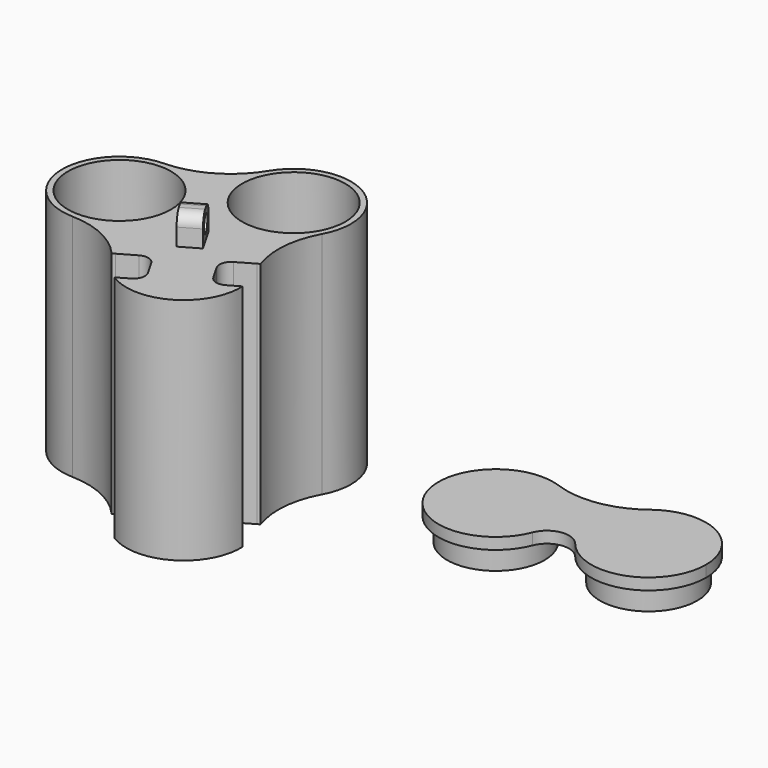
from build123d import *

# Parameters (mm, degrees)
F0_R     = 11.43
F1_DEPTH = 50.8
F2_R     = 11.43
F3_DEPTH = 48.26
F5_DEPTH = 6.35
F6_R     = 11.303
F7_DEPTH = 2.54
F8_R     = 10.795
F8_R_2   = 10.16
F9_DEPTH = 5.08
F10_R    = 2.54
F12_D    = 3.81


# Not quite as in the source:
# - a feature names something its author has since deleted; it is built from what else it names


with BuildPart() as f1:
    # F0 (on Top) → F1 (new body)
    with BuildSketch(Plane.XY):
        with BuildLine():
            ThreePointArc((-26.6880410914, -27.9366493299), (-17.5198893886, -24.3227590811), (-13.696455988, -15.239997089))
            ThreePointArc((-13.696455988, -15.239997089), (-17.5198098165, -6.1573128632), (-26.687818625, -2.5433397409))
            ThreePointArc((-26.687818625, -2.5433397409), (-39.0964559875, -15.2398858265), (-26.6880410914, -27.9366493299))
        make_face()
        with Locations((-26.396455988, -15.239997089)):
            Circle(F0_R, mode=Mode.SUBTRACT)
        with BuildLine():
            ThreePointArc((-6.3500025059, -19.4814729967), (-11.2476380181, -19.4814737375), (-13.696455988, -15.239997089))
            ThreePointArc((-13.696455988, -15.239997089), (-17.5198893886, -24.3227590811), (-26.6880410914, -27.9366493299))
            ThreePointArc((-26.6880410914, -27.9366493299), (-19.0079324117, -29.7476810857), (-12.7205570443, -34.5155754156))
            Line((-12.7205570443, -34.5155754156), (-12.1476135977, -34.1847861939))
            ThreePointArc((-12.1476135977, -34.1847861939), (-11.8147071535, -25.8213790536), (-6.3500025059, -19.4814729967))
        make_face()
        with BuildLine():
            ThreePointArc((-26.687818625, -2.5433397409), (-17.5198098165, -6.1573128632), (-13.696455988, -15.239997089))
            ThreePointArc((-13.696455988, -15.239997089), (-11.2476381845, -10.9985205365), (-6.3500028388, -10.9985209891))
            ThreePointArc((-6.3500028388, -10.9985209891), (-12.3041591128, -3.1460560273), (-10.8499450322, 6.6006585125))
            ThreePointArc((-10.8499450322, 6.6006585125), (-17.5998643999, 0.0038612886), (-26.687818625, -2.5433397409))
        make_face()
        with BuildLine():
            ThreePointArc((-6.3500028388, -10.9985209891), (-11.2476381845, -10.9985205365), (-13.696455988, -15.239997089))
            ThreePointArc((-13.696455988, -15.239997089), (-11.2476380181, -19.4814737375), (-6.3500025059, -19.4814729967))
            ThreePointArc((-6.3500025059, -19.4814729967), (-4.557344255, -17.6888142035), (-3.9011858191, -15.239997089))
            ThreePointArc((-3.9011858191, -15.239997089), (-4.5573443511, -12.791179808), (-6.3500028388, -10.9985209891))
        make_face()
        with BuildLine():
            ThreePointArc((-10.8499450322, 6.6006585125), (-12.3041591128, -3.1460560273), (-6.3500028388, -10.9985209891))
            ThreePointArc((-6.3500028388, -10.9985209891), (3.4275119235, -12.2287432721), (11.1413104344, -6.0959988356))
            ThreePointArc((11.1413104344, -6.0959988356), (12.3041586977, -3.1460576507), (12.7, 0))
            ThreePointArc((12.7, 0), (3.4275135369, 12.2287428199), (-10.8499450322, 6.6006585125))
        make_face()
        Circle(F0_R, mode=Mode.SUBTRACT)
        with BuildLine():
            ThreePointArc((11.1413104344, -6.0959988356), (3.4275119235, -12.2287432721), (-6.3500028388, -10.9985209891))
            ThreePointArc((-6.3500028388, -10.9985209891), (-4.5573443511, -12.791179808), (-3.9011858191, -15.239997089))
            ThreePointArc((-3.9011858191, -15.239997089), (-4.557344255, -17.6888142035), (-6.3500025059, -19.4814729967))
            ThreePointArc((-6.3500025059, -19.4814729967), (1.8728689002, -17.9188492428), (9.2822469769, -21.8122441204))
            Line((9.2822469769, -21.8122441204), (9.8548289521, -21.4816635945))
            ThreePointArc((9.8548289521, -21.4816635945), (8.8695235868, -13.6526593666), (11.1413104344, -6.0959988356))
        make_face()
        with BuildLine():
            ThreePointArc((9.2822469769, -21.8122441204), (1.8728689002, -17.9188492428), (-6.3500025059, -19.4814729967))
            ThreePointArc((-6.3500025059, -19.4814729967), (-11.8147071535, -25.8213790536), (-12.1476135977, -34.1847861939))
            Line((-12.1476135977, -34.1847861939), (-8.5817221083, -32.126016734))
            ThreePointArc((-8.5817221083, -32.126016734), (-6.6543217897, -31.8722692357), (-5.1120173776, -33.0557204943))
            Line((-5.1120173776, -33.0557204943), (-3.2583915378, -36.2662929918))
            ThreePointArc((-3.2583915378, -36.2662929918), (-3.0046440395, -38.1936933104), (-4.1880952981, -39.7359977225))
            Line((-4.1880952981, -39.7359977225), (-6.7686986704, -41.225910533))
            ThreePointArc((-6.7686986704, -41.225910533), (6.3500024258, -41.4785154055), (12.6905856699, -29.9910817583))
            Line((12.6905856699, -29.9910817583), (10.1099822977, -31.4809945689))
            ThreePointArc((10.1099822977, -31.4809945689), (8.1825819791, -31.7347420671), (6.640277567, -30.5512908085))
            Line((6.640277567, -30.5512908085), (4.7866517271, -27.340718311))
            ThreePointArc((4.7866517271, -27.340718311), (4.5329042289, -25.4133179924), (5.7163554875, -23.8710135804))
            Line((5.7163554875, -23.8710135804), (9.2822469769, -21.8122441204))
        make_face()
        Circle(F0_R)
        with Locations((-26.396455988, -15.239997089)):
            Circle(F0_R)
    extrude(amount=F1_DEPTH)

    # F2 (on face) → F3 (cut)
    with BuildSketch(Plane.XY.offset(50.8)):
        Circle(F2_R)
        with Locations((-26.396455988, -15.239997089)):
            Circle(F2_R)
    extrude(amount=-F3_DEPTH, mode=Mode.SUBTRACT)

    # F4 (on face) → F5 (join)
    with BuildSketch(Plane.XY.offset(50.8)):
        Polygon((-4.7208319521, -17.694307821), (-8.7123144021, -19.9987924618), (-5.5323556007, -25.5066398663), (-1.5408731507, -23.2021552255), align=None)
    extrude(amount=F5_DEPTH)

    # F10
    f10_edges = [f1.edges().sort_by_distance(p)[0] for p in [
        (-3.536614, -24.354398, 57.15),
        (-6.716573, -18.84655, 57.15),
    ]]
    fillet(f10_edges, radius=F10_R)

    # F12 (through all)
    with Locations(Plane(origin=(-15.1939675014, -8.7722456953, 0), x_dir=(0.500000191, -0.8660252935, 0), z_dir=(-0.8660252935, -0.500000191, 0))):
        with Locations((16.1432588328, 54.0085211396)):
            Hole(F12_D / 2)


with BuildPart() as f7:
    # F6 (on Top) → F7 (new body)
    with BuildSketch(Plane.XY):
        with BuildLine():
            ThreePointArc((44.0081312178, 18.3094680903), (50.0822556943, 13.6613132529), (52.3854183536, 6.367769991))
            ThreePointArc((52.3854183536, 6.367769991), (52.1684100917, 4.0300537406), (51.5248014611, 1.772227843))
            ThreePointArc((51.5248014611, 1.772227843), (55.3424694696, 4.8401671142), (59.9082168201, 3.0679392713))
            ThreePointArc((59.9082168201, 3.0679392713), (57.1989858639, 12.5428148688), (62.0815389765, 21.1028309357))
            ThreePointArc((62.0815389765, 21.1028309357), (53.401953478, 17.3955488238), (44.0081312178, 18.3094680903))
        make_face()
        with BuildLine():
            ThreePointArc((51.5248014611, 1.772227843), (52.1684100917, 4.0300537406), (52.3854183536, 6.367769991))
            ThreePointArc((52.3854183536, 6.367769991), (50.0822556943, 13.6613132529), (44.0081312178, 18.3094680903))
            ThreePointArc((44.0081312178, 18.3094680903), (28.1236963669, 1.1126215915), (51.5248014611, 1.772227843))
        make_face()
        with Locations((39.6854183536, 6.367769991)):
            Circle(F6_R, mode=Mode.SUBTRACT)
        with Locations((39.6854183536, 6.367769991)):
            Circle(F6_R)
        with BuildLine():
            ThreePointArc((82.5077646182, 11.0233747334), (75.4276816261, 22.4122523263), (62.0815389765, 21.1028309357))
            ThreePointArc((62.0815389765, 21.1028309357), (57.1989858639, 12.5428148688), (59.9082168201, 3.0679392713))
            ThreePointArc((59.9082168201, 3.0679392713), (74.0247388275, -0.9560713522), (82.5077646182, 11.0233747334))
        make_face()
        with Locations((69.8077646182, 11.0233747334)):
            Circle(F6_R, mode=Mode.SUBTRACT)
        with Locations((69.8077646182, 11.0233747334)):
            Circle(F6_R)
    extrude(amount=F7_DEPTH)

    # F8 (on face) → F9 (join)
    with BuildSketch(Plane(origin=(0, 0, 0), x_dir=(1, 0, 0), z_dir=(0, 0, -1))):
        with Locations((39.6854183536, -6.367769991)):
            Circle(F8_R)
        with Locations((39.6854183536, -6.367769991)):
            Circle(F8_R_2, mode=Mode.SUBTRACT)
        with Locations((69.8077646182, -11.0233747334)):
            Circle(F8_R)
        with Locations((69.8077646182, -11.0233747334)):
            Circle(F8_R_2, mode=Mode.SUBTRACT)
    extrude(amount=F9_DEPTH)


solid = Compound([f1.part, f7.part])
